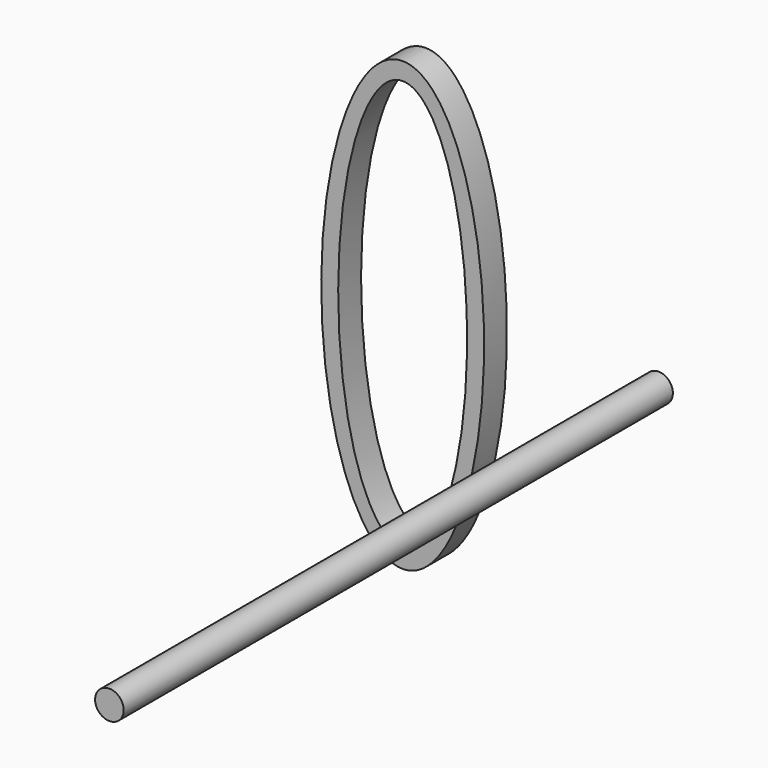
from build123d import *

# Parameters (mm, degrees)
F0_R     = 3.175
F1_DEPTH = 152.4
F3_DEPTH = 6.35


# Not quite as in the source:
# - a length typed as a fraction of an inch, garbled in the dataset ("3 / 203.2 mm" for 3/8 in), is restored


with BuildPart() as f1:
    # F0 (on Front) → F1 (new body)
    with BuildSketch(Plane.XZ):
        Circle(F0_R)
    extrude(amount=F1_DEPTH)


with BuildPart() as f3:
    # F2 (on Front) → F3 (new body)
    with BuildSketch(Plane.XZ):
        with BuildLine():
            add(Edge.make_bspline(
                [(-51.7357885838, 49.6302656829), (-83.0476053629, 49.6302656829), (-67.3916969734, -24.8151328415), (-51.7357885838, -99.2605313659), (-36.0798801942, -24.8151328415), (-20.4239718046, 49.6302656829), (-51.7357885838, 49.6302656829)],
                knots=[0, 0, 0, 2.0943951024, 2.0943951024, 4.1887902048, 4.1887902048, 6.2831853072, 6.2831853072, 6.2831853072], degree=2, weights=[1, 0.5, 1, 0.5, 1, 0.5, 1]))
        make_face()
        with BuildLine():
            add(Edge.make_bspline(
                [(-51.7357885838, 45.7200035453), (-76.5309288558, 45.7200035453), (-64.1333587198, -22.8600017726), (-51.7357885838, -91.4400070906), (-39.3382184477, -22.8600017726), (-26.9406483117, 45.7200035453), (-51.7357885838, 45.7200035453)],
                knots=[0, 0, 0, 2.0943951024, 2.0943951024, 4.1887902048, 4.1887902048, 6.2831853072, 6.2831853072, 6.2831853072], degree=2, weights=[1, 0.5, 1, 0.5, 1, 0.5, 1]))
        make_face(mode=Mode.SUBTRACT)
    extrude(amount=F3_DEPTH)


solid = Compound([f1.part, f3.part])
